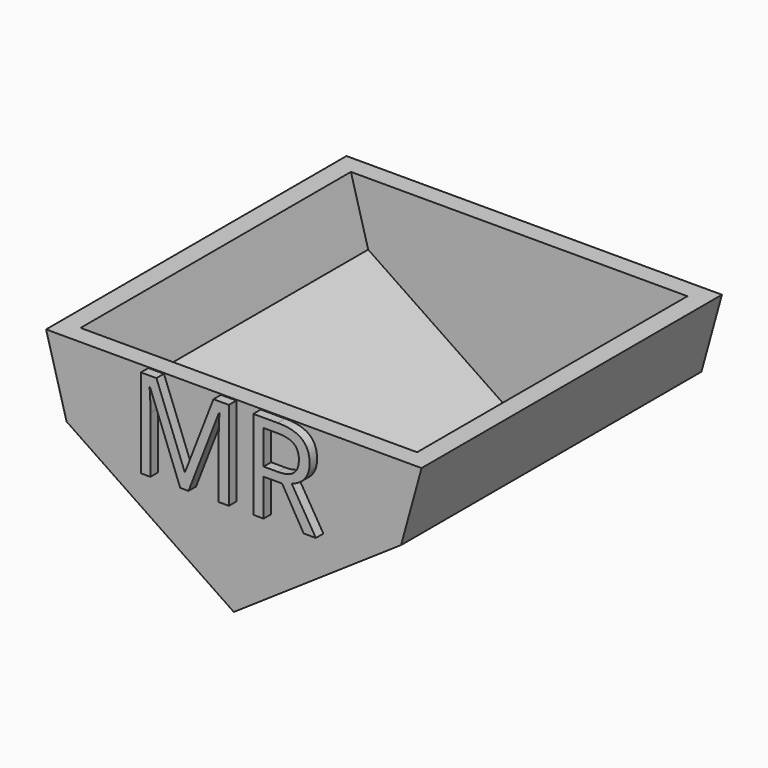
from build123d import *

# Parameters (mm, degrees)
F1_DEPTH     = 50.8
F3_DEPTH     = 59.69
F5_T         = -2.54
F6_TEXT_SIZE = 16.8405861283
F7_DEPTH     = 1.27


# Not quite as in the source:
# - a feature of the source that left no trace in its solid (it failed there, or was rolled back) is left out
# - Text() gives the source's letters only with a copy of the font that has no kerning and outlines rounded to 1/6400 em; it was checked with that copy


with BuildPart() as f1:
    # F0 (on Front) → F1 (new body)
    with BuildSketch(Plane.XZ):
        Polygon((25.4, 0), (0, 0), (0, -25.4), (22.6305667311, -10.0742522627), align=None)
        Polygon((0, -25.4), (0, 0), (-25.4, 0), (-22.6305667311, -10.0742522627), align=None)
    extrude(amount=F1_DEPTH)

    # F2 (on face) → F3 (cut)
    with BuildSketch(Plane.XY):
        Polygon((25.4, -50.8), (0, -50.8), (-25.4, -50.8), (-25.4, -37.4775226303), (-36.1447297037, -31.8418368697), (-25.4, -109.5501482487), (76.0752484202, -97.5556150079), (49.0627847612, -29.5899398625), (25.4, -39.8194669929), align=None)
    extrude(amount=-F3_DEPTH, mode=Mode.SUBTRACT)

    # F5
    f5_openings = [f1.faces().sort_by_distance(p)[0] for p in [
        (0, -25.4, 0),
    ]]
    offset(amount=F5_T, openings=f5_openings)

    # F6 (on face) → F7 (join)
    with BuildSketch(Plane.XZ.offset(50.8)):
        with Locations((-13.2093347444, -12.1252220124)):
            Text('MR', F6_TEXT_SIZE, font='Open Sans', text_align=(TextAlign.LEFT, TextAlign.BOTTOM))
    extrude(amount=F7_DEPTH)


solid = f1.part
